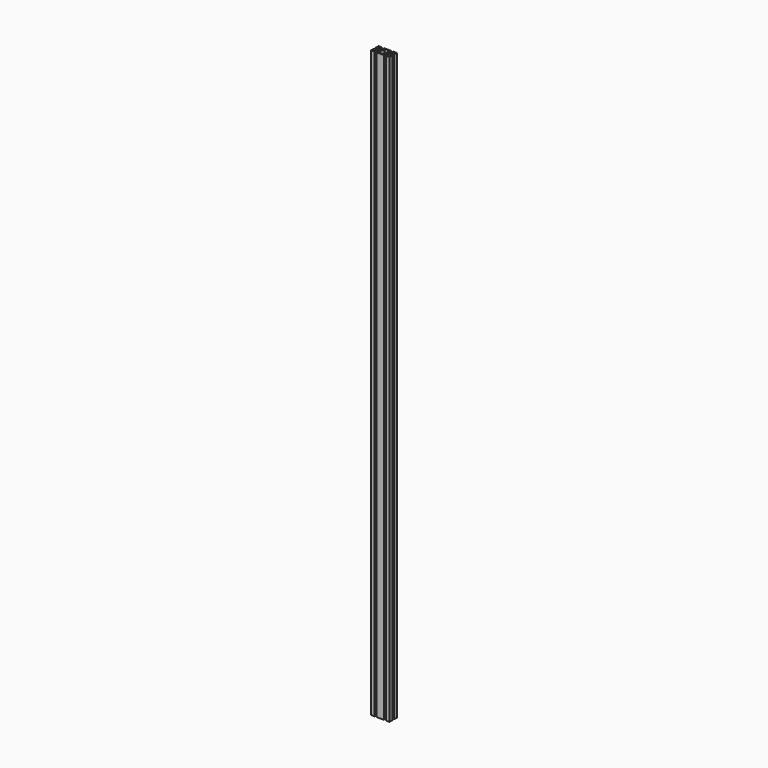
from build123d import *

# Parameters (mm, degrees)
F0_R     = 3
F0_R_2   = 2.5
F1_DEPTH = 1900
F2_R     = 2
F3_R     = 7


# Not quite as in the source:
# - a feature names something its author has since deleted; it is built from what else it names


with BuildPart() as f1:
    # F0 (on Top) → F1 (new body)
    with BuildSketch(Plane.XY):
        with BuildLine():
            Line((18.15, -15), (30, -15))
            Line((30, -15), (30, -3.15))
            Line((30, -3.15), (27.5, -3.15))
            Line((27.5, -3.15), (27.5, -5.15))
            Line((27.5, -5.15), (21.5477069044, -5.15))
            ThreePointArc((21.5477069044, -5.15), (19.5, 0), (21.5477069044, 5.15))
            Line((21.5477069044, 5.15), (27.5, 5.15))
            Line((27.5, 5.15), (27.5, 3.15))
            Line((27.5, 3.15), (30, 3.15))
            Line((30, 3.15), (30, 15))
            Line((30, 15), (18.15, 15))
            Line((18.15, 15), (18.15, 12.5))
            Line((18.15, 12.5), (20.15, 12.5))
            Line((20.15, 12.5), (20.15, 6.5477069044))
            ThreePointArc((20.15, 6.5477069044), (15, 4.5), (9.85, 6.5477069044))
            Line((9.85, 6.5477069044), (9.85, 12.5))
            Line((9.85, 12.5), (11.85, 12.5))
            Line((11.85, 12.5), (11.85, 15))
            Line((11.85, 15), (-11.85, 15))
            Line((-11.85, 15), (-11.85, 12.5))
            Line((-11.85, 12.5), (-9.85, 12.5))
            Line((-9.85, 12.5), (-9.85, 6.5477069044))
            ThreePointArc((-9.85, 6.5477069044), (-15, 4.5), (-20.15, 6.5477069044))
            Line((-20.15, 6.5477069044), (-20.15, 12.5))
            Line((-20.15, 12.5), (-18.15, 12.5))
            Line((-18.15, 12.5), (-18.15, 15))
            Line((-18.15, 15), (-30, 15))
            Line((-30, 15), (-30, 3.15))
            Line((-30, 3.15), (-27.5, 3.15))
            Line((-27.5, 3.15), (-27.5, 5.15))
            Line((-27.5, 5.15), (-21.5477069044, 5.15))
            ThreePointArc((-21.5477069044, 5.15), (-19.5, 0), (-21.5477069044, -5.15))
            Line((-21.5477069044, -5.15), (-27.5, -5.15))
            Line((-27.5, -5.15), (-27.5, -3.15))
            Line((-27.5, -3.15), (-30, -3.15))
            Line((-30, -3.15), (-30, -15))
            Line((-30, -15), (-18.15, -15))
            Line((-18.15, -15), (-18.15, -12.5))
            Line((-18.15, -12.5), (-20.15, -12.5))
            Line((-20.15, -12.5), (-20.15, -6.5477069044))
            ThreePointArc((-20.15, -6.5477069044), (-15, -4.5), (-9.85, -6.5477069044))
            Line((-9.85, -6.5477069044), (-9.85, -12.5))
            Line((-9.85, -12.5), (-11.85, -12.5))
            Line((-11.85, -12.5), (-11.85, -15))
            Line((-11.85, -15), (11.85, -15))
            Line((11.85, -15), (11.85, -12.5))
            Line((11.85, -12.5), (9.85, -12.5))
            Line((9.85, -12.5), (9.85, -6.5477069044))
            ThreePointArc((9.85, -6.5477069044), (15, -4.5), (20.15, -6.5477069044))
            Line((20.15, -6.5477069044), (20.15, -12.5))
            Line((20.15, -12.5), (18.15, -12.5))
            Line((18.15, -12.5), (18.15, -15))
        make_face()
        with Locations((-25, -10)):
            Circle(F0_R, mode=Mode.SUBTRACT)
        with Locations((25, -10)):
            Circle(F0_R, mode=Mode.SUBTRACT)
        with Locations((-15, 0)):
            Circle(F0_R_2, mode=Mode.SUBTRACT)
        with Locations((-25, 10)):
            Circle(F0_R, mode=Mode.SUBTRACT)
        Polygon((-7, 7), (-7, 12.5), (0, 12.5), (7, 12.5), (7, 7), (10, 0), (7, -7), (7, -12.5), (0, -12.5), (-7, -12.5), (-7, -7), (-10, 0), align=None, mode=Mode.SUBTRACT)
        with Locations((15, 0)):
            Circle(F0_R_2, mode=Mode.SUBTRACT)
        with Locations((25, 10)):
            Circle(F0_R, mode=Mode.SUBTRACT)
    extrude(amount=F1_DEPTH)

    # F2
    f2_edges = [f1.edges().sort_by_distance(p)[0] for p in [
        (-7, 12.5, 950),
        (7, 12.5, 950),
    ]]
    fillet(f2_edges, radius=F2_R)

    # F3
    f3_edges = [f1.edges().sort_by_distance(p)[0] for p in [
        (-7, 7, 950),
        (-10, 0, 950),
        (7, 7, 950),
        (10, 0, 950),
    ]]
    fillet(f3_edges, radius=F3_R)


solid = f1.part
